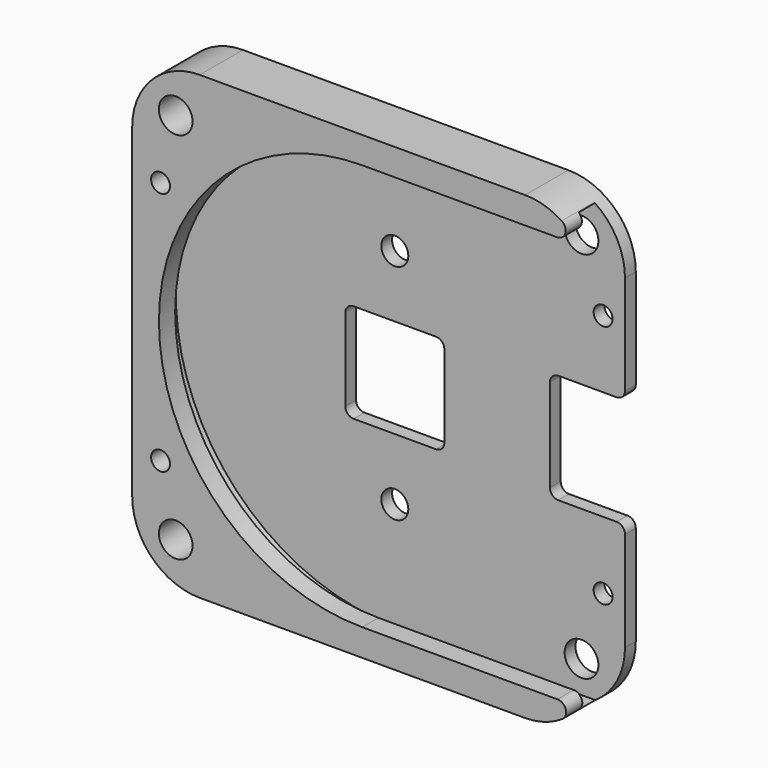
from build123d import *

# Parameters (mm, degrees)
F0_W         = 43.307
F0_H         = 43.307
F1_DEPTH     = 1.27
F3_DEPTH     = 3.175
F5_DEPTH     = 1.905
F6_R         = 0.889
F7_DEPTH     = 5.081
F8_W         = 9.3218
F8_H         = 9.3218
F8_W_2       = 7.0612
F8_H_2       = 10.3124
F10_DEPTH    = 1.27
F11_D        = 3.175
F14_D        = 2.54
F15_R        = 6.35
F16_T4_DEPTH = 12.7851645967
F16_T9_DEPTH = 12.8907938144
F17_R        = 0.7874
F18_D        = 3.175
F18_DEPTH    = 3.175
F18_TIP      = 0.9538662327


# Not quite as in the source:
# - a fillet or chamfer that OpenCascade refuses, or shapes differently, is made with other operations: its cross-section is extruded or revolved along the edge and cut away or added


with BuildPart() as f1:
    # F0 (on Front) → F1 (new body)
    with BuildSketch(Plane.XZ):
        with Locations((21.6535, 21.6535)):
            Rectangle(F0_W, F0_H)
    extrude(amount=F1_DEPTH)

    # F2 (on Front) → F3 (join)
    with BuildSketch(Plane.XZ):
        with BuildLine():
            Line((43.307, 43.307), (0, 43.307))
            Line((0, 43.307), (0, 0))
            Line((0, 0), (43.307, 0))
            Line((43.307, 0), (43.307, 1.0922))
            Line((43.307, 1.0922), (21.6408, 1.0922))
            ThreePointArc((21.6408, 1.0922), (1.0668, 21.6662), (21.6408, 42.2402))
            Line((21.6408, 42.2402), (43.307, 42.2402))
            Line((43.307, 42.2402), (43.307, 43.307))
        make_face()
    extrude(amount=F3_DEPTH)

    # F4 (on face) → F5 (join)
    with BuildSketch(Plane.XZ.offset(3.175)):
        with BuildLine():
            Line((43.307, 43.307), (0, 43.307))
            Line((0, 43.307), (0, 0))
            Line((0, 0), (43.307, 0))
            Line((43.307, 0), (43.307, 2.54))
            Line((43.307, 2.54), (21.6408, 2.54))
            ThreePointArc((21.6408, 2.54), (2.5146, 21.6662), (21.6408, 40.7924))
            Line((21.6408, 40.7924), (43.307, 40.7924))
            Line((43.307, 40.7924), (43.307, 43.307))
        make_face()
    extrude(amount=F5_DEPTH)

    # F6 (on face) → F7 (cut, through all)
    with BuildSketch(Plane(origin=(0, 0, 0), x_dir=(-1, 0, 0), z_dir=(0, 1, 0))):
        with Locations((-41.2496, 33.1724)):
            Circle(F6_R)
        with Locations((-2.667, 33.1724)):
            Circle(F6_R)
        with Locations((-41.2496, 10.16)):
            Circle(F6_R)
        with Locations((-2.667, 10.16)):
            Circle(F6_R)
    extrude(amount=-F7_DEPTH, mode=Mode.SUBTRACT)

    # F8 (on face) → F10 (cut, through all)
    with BuildSketch(Plane.XZ.offset(1.27)):
        with Locations((21.6535, 21.6535)):
            Rectangle(F8_W, F8_H)
        with Locations((39.7764, 21.6662)):
            Rectangle(F8_W_2, F8_H_2)
    extrude(amount=-F10_DEPTH, mode=Mode.SUBTRACT)

    # F11 (through all)
    with Locations(Plane(origin=(0, 0, 0), x_dir=(-1, 0, 0), z_dir=(0, 1, 0))):
        with Locations((-4.0894, 39.2176), (-4.0894, 4.0894)):
            Hole(F11_D / 2)

    # F14 (through all)
    with Locations(Plane(origin=(0, 0, 0), x_dir=(-1, 0, 0), z_dir=(0, 1, 0))):
        with Locations((-21.6535, 32.1564), (-21.6535, 11.176)):
            Hole(F14_D / 2)

    # F15
    f15_edges = [f1.edges().sort_by_distance(p)[0] for p in [
        (0, -2.54, 43.307),
        (43.307, -2.54, 43.307),
        (43.307, -2.54, 0),
        (0, -2.54, 0),
    ]]
    fillet(f15_edges, radius=F15_R)

    # F16: fillet of radius 0.8128 on 2 edges, made by hand


with BuildPart() as f16_tool2:
    # F16_s3 → F16_t4 (new body)
    with BuildSketch(Plane.XZ.offset(10.5200822984)):
        with BuildLine():
            ThreePointArc((40.005, 2.54), (40.7835212046, 1.9607563614), (40.452412844, 1.0486238532))
            ThreePointArc((40.452412844, 1.0486238532), (41.3090658387, 1.7259300464), (42.037, 2.54))
            Line((42.037, 2.54), (40.005, 2.54))
        make_face()
    extrude(amount=-F16_T4_DEPTH)

    split(bisect_by=Plane.XZ.offset(1.27), keep=Keep.TOP)


with BuildPart() as f1_1:
    add(f1.part)

    # F16_t1: cut F16_tool2
    add(f16_tool2.part, mode=Mode.SUBTRACT)


with BuildPart() as f16_tool7:
    # F16_s8 → F16_t9 (new body)
    with BuildSketch(Plane.XZ.offset(10.5728969072)):
        with BuildLine():
            ThreePointArc((39.9661228955, 40.7924), (40.7456166441, 41.374910322), (40.4078290086, 42.2875045872))
            ThreePointArc((40.4078290086, 42.2875045872), (41.2779959557, 41.6101165847), (42.0178504068, 40.7924))
            Line((42.0178504068, 40.7924), (39.9661228955, 40.7924))
        make_face()
    extrude(amount=-F16_T9_DEPTH)

    split(bisect_by=Plane.XZ.offset(1.27), keep=Keep.TOP)


with BuildPart() as f1_2:
    add(f1_1.part)

    # F16_t6: cut F16_tool7
    add(f16_tool7.part, mode=Mode.SUBTRACT)

    # F17
    f17_edges = [f1_2.edges().sort_by_distance(p)[0] for p in [
        (43.307, -0.635, 26.8224),
        (36.2458, -0.635, 26.8224),
        (16.9926, -0.635, 26.3144),
        (16.9926, -0.635, 16.9926),
        (26.3144, -0.635, 16.9926),
        (43.307, -0.635, 16.51),
        (36.2458, -0.635, 16.51),
        (26.3144, -0.635, 26.3144),
    ]]
    fillet(f17_edges, radius=F17_R)

    # F18
    with Locations(Plane(origin=(0, 0, 0), x_dir=(-1, 0, 0), z_dir=(0, 1, 0))):
        with Locations((-39.2176, 4.0894), (-39.2176, 39.2176)):
            Hole(F18_D / 2, depth=F18_DEPTH)
            with Locations((0, 0, -(F18_DEPTH + F18_TIP / 2))):  # 118° drill point
                Cone(0, F18_D / 2, F18_TIP, mode=Mode.SUBTRACT)


solid = f1_2.part
